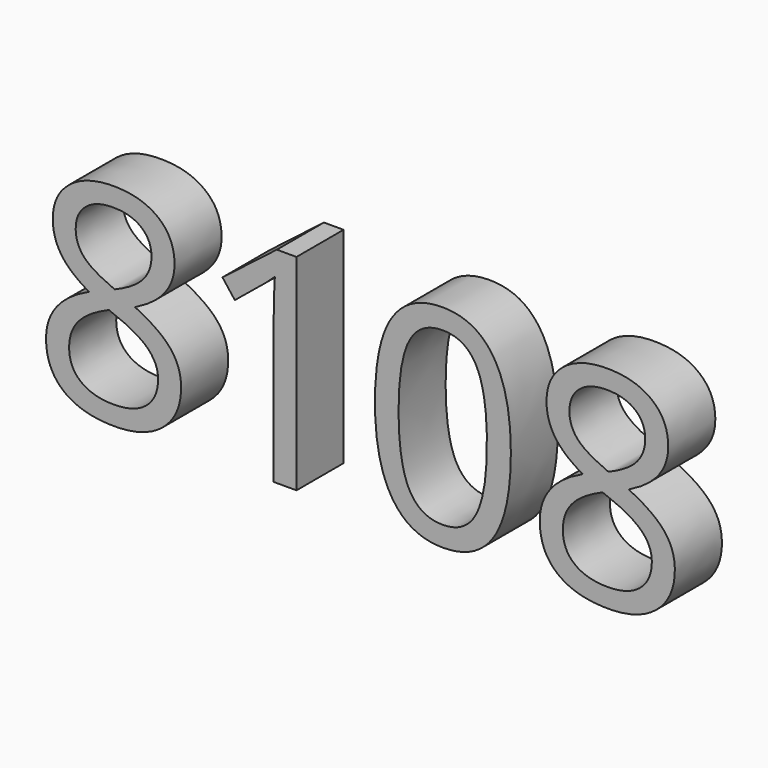
from build123d import *

# Parameters (mm, degrees)
F0_TEXT_SIZE = 124.2391304348
F1_DEPTH     = 25.4


# Not quite as in the source:
# - Text() gives the source's letters only with a copy of the font that has no kerning and outlines rounded to 1/6400 em; it was checked with that copy


with BuildPart() as f1:
    # F0 (on Front) → F1 (new body)
    with BuildSketch(Plane.XZ):
        with Locations((-205.7100122946, -35.4792188223)):
            Text('8108', F0_TEXT_SIZE, font='Open Sans', text_align=(TextAlign.LEFT, TextAlign.BOTTOM))
    extrude(amount=F1_DEPTH)


solid = f1.part
